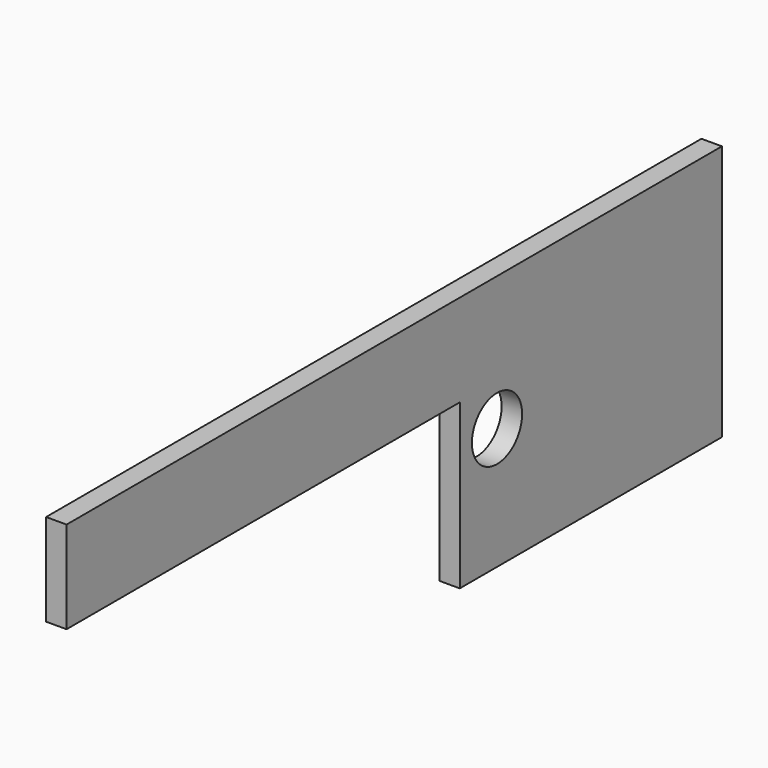
from build123d import *

# Parameters (mm, degrees)
F1_W     = 50.8
F1_H     = 25.4
F1_R     = 4.8652202412
F2_DEPTH = 3.175


# Not quite as in the source:
# - a variable given as a bare number and used for a length is read in inches; the dataset says mm whatever the document's units were


with BuildPart() as f2:
    # F1 (on Right) → F2 (new body)
    with BuildSketch(Plane.YZ):
        Polygon((63.5, 7.14375), (-63.5, 7.14375), (-63.5, -7.14375), (12.7, -7.14375), (63.5, -7.14375), align=None)
        with Locations((38.1, -19.84375)):
            Rectangle(F1_W, F1_H)
        with Locations((19.9129190296, -13.6523451656)):
            Circle(F1_R, mode=Mode.SUBTRACT)
    extrude(amount=-F2_DEPTH)


solid = f2.part
